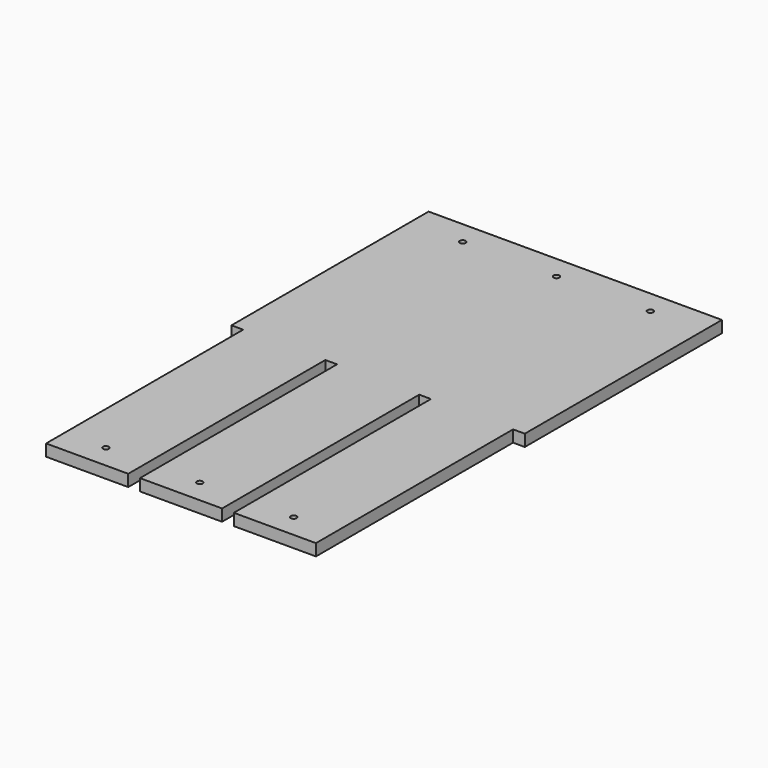
from build123d import *

# Parameters (mm, degrees)
F0_W     = 22.225
F0_H     = 120.65
F1_DEPTH = 6.35
F3_D     = 3.175


# Not quite as in the source:
# - a feature names something its author has since deleted; it is built from what else it names


with BuildPart() as f1:
    # F0 (on Top) → F1 (new body)
    with BuildSketch(Plane.XY):
        Polygon((73.025, 133.35), (-73.025, 133.35), (-73.025, 120.65), (-50.8, 120.65), (0, 120.65), (50.8, 120.65), (73.025, 120.65), align=None)
        Polygon((-50.8, -120.65), (-73.025, -120.65), (-73.025, -133.35), (-28.575, -133.35), (-28.575, -120.65), align=None)
        Polygon((73.025, -133.35), (73.025, -120.65), (50.8, -120.65), (28.575, -120.65), (28.575, -133.35), align=None)
        with Locations((-61.9125, 60.325)):
            Rectangle(F0_W, F0_H)
        with Locations((-61.9125, -60.325)):
            Rectangle(F0_W, F0_H)
        with Locations((61.9125, 60.325)):
            Rectangle(F0_W, F0_H)
        with Locations((61.9125, -60.325)):
            Rectangle(F0_W, F0_H)
        Polygon((50.8, 0), (50.8, 120.65), (0, 120.65), (0, 0), (22.225, 0), (28.575, 0), align=None)
        Polygon((22.225, -120.65), (0, -120.65), (-22.225, -120.65), (-22.225, -133.35), (22.225, -133.35), align=None)
        Polygon((0, 120.65), (-50.8, 120.65), (-50.8, 0), (-28.575, 0), (-22.225, 0), (0, 0), align=None)
        with Locations((-39.6875, -60.325)):
            Rectangle(F0_W, F0_H)
        with Locations((-11.1125, -60.325)):
            Rectangle(F0_W, F0_H)
        with Locations((11.1125, -60.325)):
            Rectangle(F0_W, F0_H)
        with Locations((39.6875, -60.325)):
            Rectangle(F0_W, F0_H)
        Polygon((79.375, 133.35), (73.025, 133.35), (73.025, 120.65), (73.025, 0), (79.375, 0), align=None)
        Polygon((-73.025, 120.65), (-73.025, 133.35), (-79.375, 133.35), (-79.375, 0), (-73.025, 0), align=None)
    extrude(amount=F1_DEPTH)

    # F3 (through all)
    with Locations(Plane.XY.offset(6.35)):
        with Locations((-50.8, 120.65), (0, 120.65), (50.8, 120.65), (50.8, -120.65), (0, -120.65), (-50.8, -120.65)):
            Hole(F3_D / 2)


solid = f1.part
